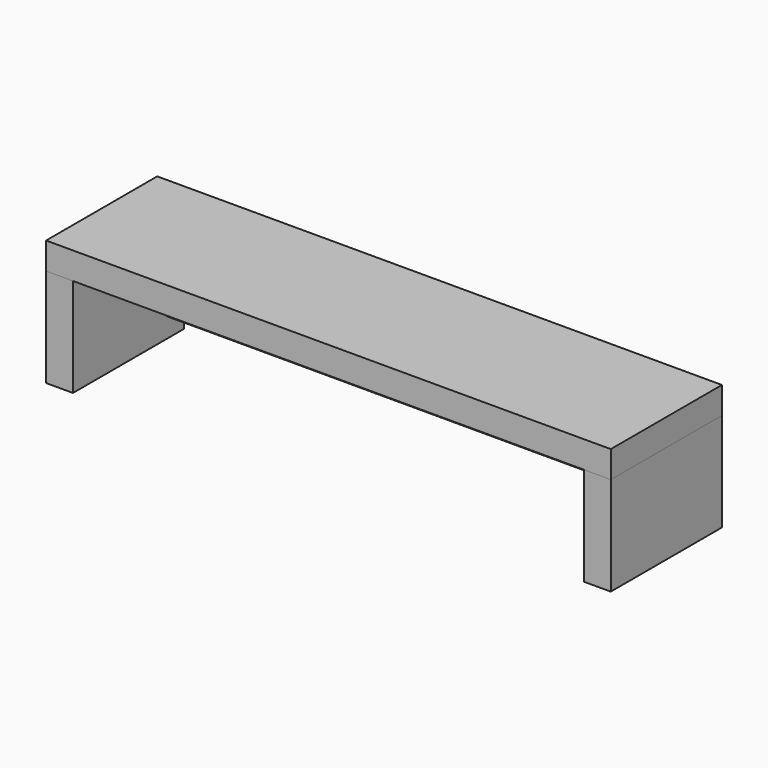
from build123d import *

# Parameters (mm, degrees)
F0_W        = 400.05
F0_H        = 98.425
F1_DEPTH    = 19.05
F2_W        = 19.05
F2_H        = 98.425
F3_DEPTH    = 69.85
F4_W        = 9.525
F4_H        = 19.05
F5_DEPTH    = 361.95
F6_T1_DEPTH = 387.35


# Not quite as in the source:
# - a fillet or chamfer that OpenCascade refuses, or shapes differently, is made with other operations: its cross-section is extruded or revolved along the edge and cut away or added


with BuildPart() as f1:
    # F0 (on Top) → F1 (new body)
    with BuildSketch(Plane.XY):
        with Locations((-200.025, -49.2125)):
            Rectangle(F0_W, F0_H)
    extrude(amount=-F1_DEPTH)


with BuildPart() as f3:
    # F2 (on face) → F3 (new body)
    with BuildSketch(Plane(origin=(0, 0, -19.05), x_dir=(1, 0, 0), z_dir=(0, 0, -1))):
        with Locations((-9.525, 49.2125)):
            Rectangle(F2_W, F2_H)
    extrude(amount=F3_DEPTH)


with BuildPart() as f3b:
    # F2 (on face) → F3, piece 2 (new body)
    with BuildSketch(Plane(origin=(0, 0, -19.05), x_dir=(1, 0, 0), z_dir=(0, 0, -1))):
        with Locations((-390.525, 49.2125)):
            Rectangle(F2_W, F2_H)
    extrude(amount=F3_DEPTH)


with BuildPart() as f5:
    # F4 (on face) → F5 (new body, through all)
    with BuildSketch(Plane.YZ.offset(-381)):
        with Locations((-11.8602966547, -66.8099847376)):
            Rectangle(F4_W, F4_H)
    extrude(amount=F5_DEPTH)

    # F6: fillet of radius 5.08 on 4 edges, made by hand

    # F6_s2 → F6_t1 (cut)
    with BuildSketch(Plane.YZ.offset(-393.7)):
        with BuildLine():
            ThreePointArc((-11.5427966547, -76.3349847376), (-15.1348991031, -74.8470871861), (-16.6227966547, -71.2549847376))
            Line((-16.6227966547, -71.2549847376), (-16.6227966547, -76.3349847376))
            Line((-16.6227966547, -76.3349847376), (-11.5427966547, -76.3349847376))
        make_face()
        with BuildLine():
            ThreePointArc((-12.1777966547, -76.3349847376), (-8.5856942063, -74.8470871861), (-7.0977966547, -71.2549847376))
            Line((-7.0977966547, -71.2549847376), (-7.0977966547, -76.3349847376))
            Line((-7.0977966547, -76.3349847376), (-12.1777966547, -76.3349847376))
        make_face()
        with BuildLine():
            ThreePointArc((-11.5427966547, -57.2849847376), (-15.1348991031, -58.7728822892), (-16.6227966547, -62.3649847376))
            Line((-16.6227966547, -62.3649847376), (-16.6227966547, -57.2849847376))
            Line((-16.6227966547, -57.2849847376), (-11.5427966547, -57.2849847376))
        make_face()
        with BuildLine():
            ThreePointArc((-7.0977966547, -62.3649847376), (-8.5856942063, -58.7728822892), (-12.1777966547, -57.2849847376))
            Line((-12.1777966547, -57.2849847376), (-7.0977966547, -57.2849847376))
            Line((-7.0977966547, -57.2849847376), (-7.0977966547, -62.3649847376))
        make_face()
    extrude(amount=F6_T1_DEPTH, mode=Mode.SUBTRACT)


solid = Compound([f1.part, f3.part, f3b.part, f5.part])
